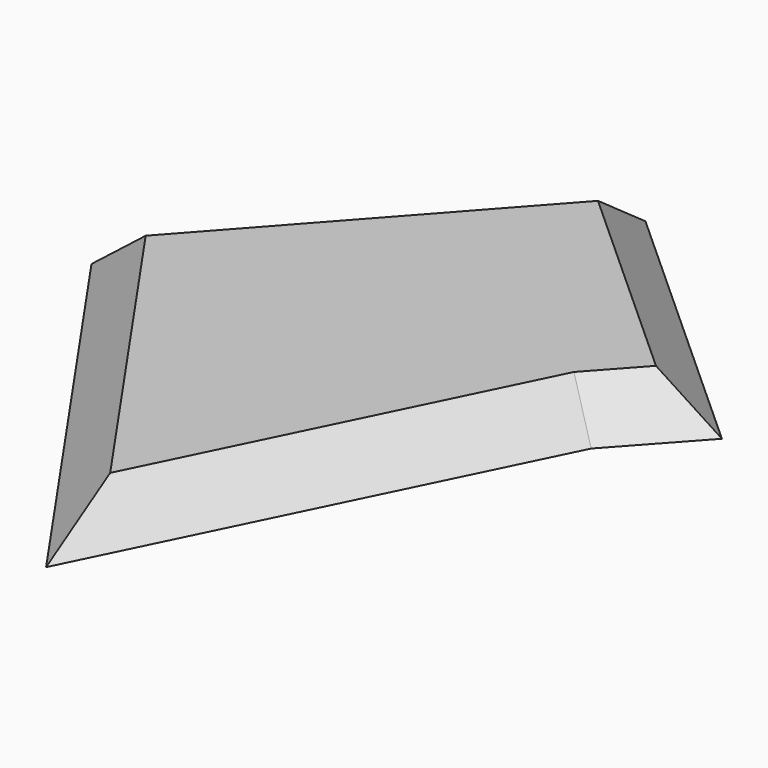
from build123d import *

# Parameters (mm, degrees)
F1_DEPTH = 5
F2_SIZE  = 4.99999


# Not quite as in the source:
# - a fillet or chamfer is up to 0.001 mm smaller than in the source, because OpenCascade refuses the exact size


with BuildPart() as f1:
    # F0 (on Top) → F1 (new body)
    with BuildSketch(Plane.XY):
        Polygon((30.7894008997, 21.0974273146), (0, 48.9359102053), (-32.5954880442, 12.5505877659), (0, -34.514117986), (23.0617076159, 12.5505877659), align=None)
    extrude(amount=F1_DEPTH)

    # F2 (size 5 in the source; OpenCascade refuses exactly that, so slightly less here)
    f2_edges = [f1.edges().sort_by_distance(p)[0] for p in [
        (-16.297744, 30.743249, 5),
        (-16.297744, -10.981765, 5),
        (11.530854, -10.981765, 5),
        (26.925554, 16.824008, 5),
        (15.3947, 35.016669, 5),
    ]]
    chamfer(f2_edges, length=F2_SIZE)


solid = f1.part
